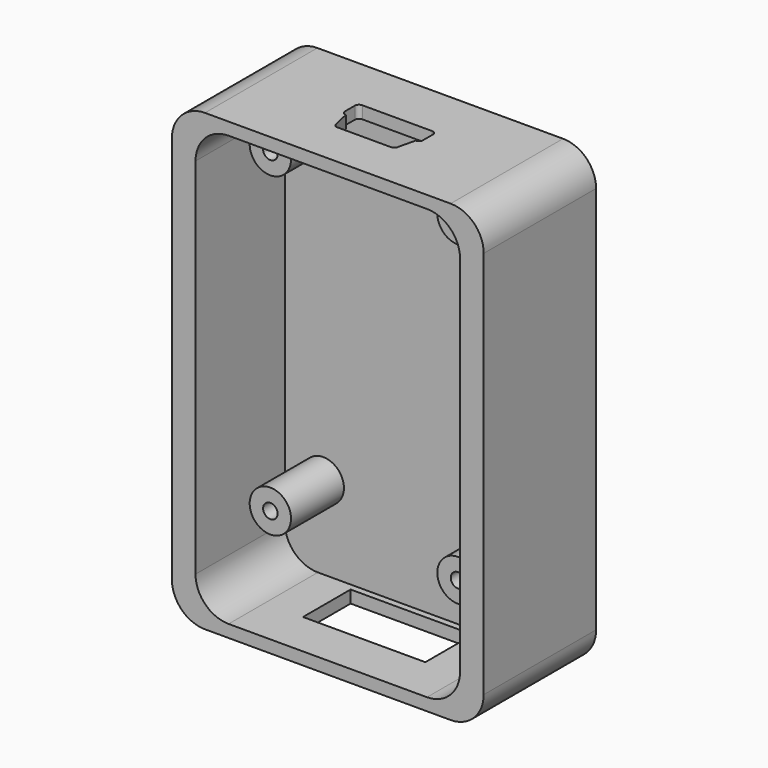
from build123d import *

# Parameters (mm, degrees)
F0_R          = 2.5
F0_R_2        = 0.875
F1_DEPTH      = 2.5
F2_DEPTH      = 16
F3_DEPTH      = 10.5
F4_DEPTH      = 1
F6_DEPTH      = 25
F7_W          = 14.8
F7_H          = 7.2
F8_DEPTH      = 25
F11_START     = 5
F10_TEXT_SIZE = 11.3789245994
F11_DEPTH     = 4


# Not quite as in the source:
# - Text() gives the source's letters only with a copy of the font that has no kerning and outlines rounded to 1/6400 em; it was checked with that copy


with BuildPart() as f1:
    # F0 (on Front) → F1 (new body)
    with BuildSketch(Plane.XZ):
        with BuildLine():
            Line((-12, -26), (0, -26))
            Line((0, -26), (0, 26))
            Line((0, 26), (-12, 26))
            ThreePointArc((-12, 26), (-14.8284271247, 24.8284271247), (-16, 22))
            Line((-16, 22), (-16, -22))
            ThreePointArc((-16, -22), (-14.8284271247, -24.8284271247), (-12, -26))
        make_face()
        with Locations((-11.35, -16)):
            Circle(F0_R, mode=Mode.SUBTRACT)
        with Locations((-11.35, 22.25)):
            Circle(F0_R, mode=Mode.SUBTRACT)
        with BuildLine():
            Line((0, -26), (12, -26))
            ThreePointArc((12, -26), (14.8284271247, -24.8284271247), (16, -22))
            Line((16, -22), (16, 22))
            ThreePointArc((16, 22), (14.8284271247, 24.8284271247), (12, 26))
            Line((12, 26), (0, 26))
            Line((0, 26), (0, -26))
        make_face()
        with Locations((11.35, -16)):
            Circle(F0_R, mode=Mode.SUBTRACT)
        with Locations((11.35, 22.25)):
            Circle(F0_R, mode=Mode.SUBTRACT)
        with BuildLine():
            Line((0, -27.5), (0, -26))
            Line((0, -26), (-12, -26))
            ThreePointArc((-12, -26), (-14.8284271247, -24.8284271247), (-16, -22))
            Line((-16, -22), (-16, 22))
            ThreePointArc((-16, 22), (-14.8284271247, 24.8284271247), (-12, 26))
            Line((-12, 26), (0, 26))
            Line((0, 26), (0, 27.5))
            Line((0, 27.5), (-14.8588332385, 27.5))
            ThreePointArc((-14.8588332385, 27.5), (-17.6872603632, 26.3284271247), (-18.8588332385, 23.5))
            Line((-18.8588332385, 23.5), (-18.8588332385, -23.5))
            ThreePointArc((-18.8588332385, -23.5), (-17.6872603632, -26.3284271247), (-14.8588332385, -27.5))
            Line((-14.8588332385, -27.5), (0, -27.5))
        make_face()
        with BuildLine():
            ThreePointArc((16, -22), (14.8284271247, -24.8284271247), (12, -26))
            Line((12, -26), (0, -26))
            Line((0, -26), (0, -27.5))
            Line((0, -27.5), (14.8588332385, -27.5))
            ThreePointArc((14.8588332385, -27.5), (17.6872603632, -26.3284271247), (18.8588332385, -23.5))
            Line((18.8588332385, -23.5), (18.8588332385, 23.5))
            ThreePointArc((18.8588332385, 23.5), (17.6872603632, 26.3284271247), (14.8588332385, 27.5))
            Line((14.8588332385, 27.5), (0, 27.5))
            Line((0, 27.5), (0, 26))
            Line((0, 26), (12, 26))
            ThreePointArc((12, 26), (14.8284271247, 24.8284271247), (16, 22))
            Line((16, 22), (16, -22))
        make_face()
        with Locations((11.35, 22.25)):
            Circle(F0_R)
        with Locations((11.35, 22.25)):
            Circle(F0_R_2, mode=Mode.SUBTRACT)
        with Locations((-11.35, 22.25)):
            Circle(F0_R)
        with Locations((-11.35, 22.25)):
            Circle(F0_R_2, mode=Mode.SUBTRACT)
        with Locations((-11.35, -16)):
            Circle(F0_R)
        with Locations((-11.35, -16)):
            Circle(F0_R_2, mode=Mode.SUBTRACT)
        with Locations((11.35, -16)):
            Circle(F0_R)
        with Locations((11.35, -16)):
            Circle(F0_R_2, mode=Mode.SUBTRACT)
        with Locations((-11.35, 22.25)):
            Circle(F0_R_2)
        with Locations((11.35, 22.25)):
            Circle(F0_R_2)
        with Locations((-11.35, -16)):
            Circle(F0_R_2)
        with Locations((11.35, -16)):
            Circle(F0_R_2)
    extrude(amount=F1_DEPTH)

    # F0 (on Front) → F2 (join)
    with BuildSketch(Plane.XZ):
        with BuildLine():
            Line((0, -27.5), (0, -26))
            Line((0, -26), (-12, -26))
            ThreePointArc((-12, -26), (-14.8284271247, -24.8284271247), (-16, -22))
            Line((-16, -22), (-16, 22))
            ThreePointArc((-16, 22), (-14.8284271247, 24.8284271247), (-12, 26))
            Line((-12, 26), (0, 26))
            Line((0, 26), (0, 27.5))
            Line((0, 27.5), (-14.8588332385, 27.5))
            ThreePointArc((-14.8588332385, 27.5), (-17.6872603632, 26.3284271247), (-18.8588332385, 23.5))
            Line((-18.8588332385, 23.5), (-18.8588332385, -23.5))
            ThreePointArc((-18.8588332385, -23.5), (-17.6872603632, -26.3284271247), (-14.8588332385, -27.5))
            Line((-14.8588332385, -27.5), (0, -27.5))
        make_face()
        with BuildLine():
            ThreePointArc((16, -22), (14.8284271247, -24.8284271247), (12, -26))
            Line((12, -26), (0, -26))
            Line((0, -26), (0, -27.5))
            Line((0, -27.5), (14.8588332385, -27.5))
            ThreePointArc((14.8588332385, -27.5), (17.6872603632, -26.3284271247), (18.8588332385, -23.5))
            Line((18.8588332385, -23.5), (18.8588332385, 23.5))
            ThreePointArc((18.8588332385, 23.5), (17.6872603632, 26.3284271247), (14.8588332385, 27.5))
            Line((14.8588332385, 27.5), (0, 27.5))
            Line((0, 27.5), (0, 26))
            Line((0, 26), (12, 26))
            ThreePointArc((12, 26), (14.8284271247, 24.8284271247), (16, 22))
            Line((16, 22), (16, -22))
        make_face()
    extrude(amount=F2_DEPTH)

    # F0 (on Front) → F3 (join)
    with BuildSketch(Plane.XZ):
        with Locations((11.35, 22.25)):
            Circle(F0_R)
        with Locations((11.35, 22.25)):
            Circle(F0_R_2, mode=Mode.SUBTRACT)
        with Locations((-11.35, 22.25)):
            Circle(F0_R)
        with Locations((-11.35, 22.25)):
            Circle(F0_R_2, mode=Mode.SUBTRACT)
        with Locations((-11.35, -16)):
            Circle(F0_R)
        with Locations((-11.35, -16)):
            Circle(F0_R_2, mode=Mode.SUBTRACT)
        with Locations((11.35, -16)):
            Circle(F0_R)
        with Locations((11.35, -16)):
            Circle(F0_R_2, mode=Mode.SUBTRACT)
    extrude(amount=F3_DEPTH)

    # F0 (on Front) → F4 (join)
    with BuildSketch(Plane.XZ):
        with BuildLine():
            Line((0, -27.5), (0, -26))
            Line((0, -26), (-12, -26))
            ThreePointArc((-12, -26), (-14.8284271247, -24.8284271247), (-16, -22))
            Line((-16, -22), (-16, 22))
            ThreePointArc((-16, 22), (-14.8284271247, 24.8284271247), (-12, 26))
            Line((-12, 26), (0, 26))
            Line((0, 26), (0, 27.5))
            Line((0, 27.5), (-14.8588332385, 27.5))
            ThreePointArc((-14.8588332385, 27.5), (-17.6872603632, 26.3284271247), (-18.8588332385, 23.5))
            Line((-18.8588332385, 23.5), (-18.8588332385, -23.5))
            ThreePointArc((-18.8588332385, -23.5), (-17.6872603632, -26.3284271247), (-14.8588332385, -27.5))
            Line((-14.8588332385, -27.5), (0, -27.5))
        make_face()
        with BuildLine():
            ThreePointArc((16, -22), (14.8284271247, -24.8284271247), (12, -26))
            Line((12, -26), (0, -26))
            Line((0, -26), (0, -27.5))
            Line((0, -27.5), (14.8588332385, -27.5))
            ThreePointArc((14.8588332385, -27.5), (17.6872603632, -26.3284271247), (18.8588332385, -23.5))
            Line((18.8588332385, -23.5), (18.8588332385, 23.5))
            ThreePointArc((18.8588332385, 23.5), (17.6872603632, 26.3284271247), (14.8588332385, 27.5))
            Line((14.8588332385, 27.5), (0, 27.5))
            Line((0, 27.5), (0, 26))
            Line((0, 26), (12, 26))
            ThreePointArc((12, 26), (14.8284271247, 24.8284271247), (16, 22))
            Line((16, 22), (16, -22))
        make_face()
    extrude(amount=-F4_DEPTH)

    # F5 (on face) → F6 (cut)
    with BuildSketch(Plane.XY.offset(27.5)):
        with BuildLine():
            Line((-3.25, -10.5), (3.25, -10.5))
            ThreePointArc((3.25, -10.5), (3.6035533906, -10.3535533906), (3.75, -10))
            Line((3.75, -10), (4.2260308638, -8))
            ThreePointArc((4.2260308638, -8), (4.5795842544, -7.8535533906), (4.7260308638, -7.5))
            Line((4.7260308638, -7.5), (4.7260308638, -6))
            ThreePointArc((4.7260308638, -6), (4.5795842544, -5.6464466094), (4.2260308638, -5.5))
            Line((4.2260308638, -5.5), (-4.2260308638, -5.5))
            ThreePointArc((-4.2260308638, -5.5), (-4.5795842544, -5.6464466094), (-4.7260308638, -6))
            Line((-4.7260308638, -6), (-4.7260308638, -7.5))
            ThreePointArc((-4.7260308638, -7.5), (-4.5795842544, -7.8535533906), (-4.2260308638, -8))
            Line((-4.2260308638, -8), (-3.75, -10))
            ThreePointArc((-3.75, -10), (-3.6035533906, -10.3535533906), (-3.25, -10.5))
        make_face()
    extrude(amount=-F6_DEPTH, mode=Mode.SUBTRACT)

    # F7 (on face) → F8 (cut)
    with BuildSketch(Plane(origin=(0, 0, -27.5), x_dir=(1, 0, 0), z_dir=(0, 0, -1))):
        with Locations((0, 6.9)):
            Rectangle(F7_W, F7_H)
    extrude(amount=-F8_DEPTH, mode=Mode.SUBTRACT)

    # F10 (on face) → F11 (join)
    with BuildSketch(Plane(origin=(0, -7.5, 0), x_dir=(-1, 0, 0), z_dir=(0, 1, 0)).offset(F11_START)):
        with Locations(Location((4.0986621752, -22.7027325328), (0, 0, 90))):
            Text('ISO-USB', F10_TEXT_SIZE, font='Open Sans', font_style=FontStyle.BOLD, text_align=(TextAlign.LEFT, TextAlign.BOTTOM))
    extrude(amount=F11_DEPTH)


solid = f1.part
